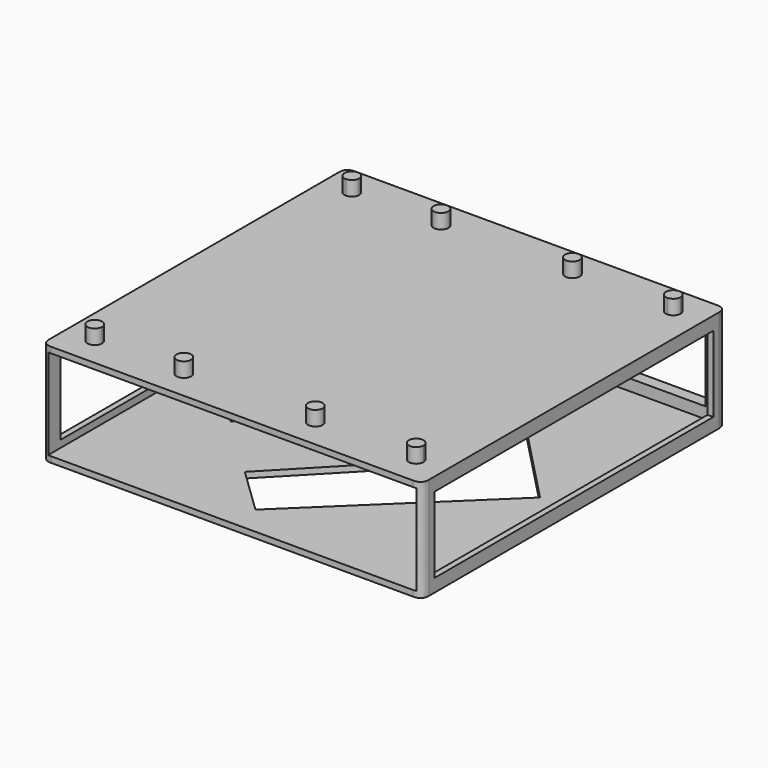
from build123d import *

# Parameters (mm, degrees)
F0_W         = 130
F0_H         = 130
F1_DEPTH     = 17.5
F2_W         = 126
F2_H         = 31
F3_DEPTH     = 126
F5_DEPTH     = 5
F7_DEPTH     = 3
F9_W         = 122.3782406645
F9_H         = 23.2565429012
F10_DEPTH    = 7
F8_W         = 119.2743226562
F8_H         = 26.0036256061
F11_DEPTH    = 130
F12_T1_DEPTH = 50


# Not quite as in the source:
# - a fillet or chamfer that OpenCascade refuses, or shapes differently, is made with other operations: its cross-section is extruded or revolved along the edge and cut away or added


with BuildPart() as f1:
    # F0 (on Top) → F1 (new body, symmetric)
    with BuildSketch(Plane.XY):
        with Locations((2.0031377077, 1.1643140912)):
            Rectangle(F0_W, F0_H)
    extrude(amount=F1_DEPTH, both=True)

    # F2 (on face) → F3 (cut)
    with BuildSketch(Plane.XZ.offset(63.8356859088)):
        with Locations((2.0031377077, 0)):
            Rectangle(F2_W, F2_H)
    extrude(amount=-F3_DEPTH, mode=Mode.SUBTRACT)

    # F4 (on face) → F5 (join)
    with BuildSketch(Plane.XY.offset(17.5)):
        with BuildLine():
            Line((-24.9968622923, -53.8356859088), (-19.9968622923, -53.8356859088))
            ThreePointArc((-19.9968622923, -53.8356859088), (-22.4968622923, -51.3356859088), (-24.9968622923, -53.8356859088))
        make_face()
        with BuildLine():
            ThreePointArc((-24.9968622923, -53.8356859088), (-22.4968622923, -56.3356859088), (-19.9968622923, -53.8356859088))
            Line((-19.9968622923, -53.8356859088), (-24.9968622923, -53.8356859088))
        make_face()
        with BuildLine():
            ThreePointArc((-19.9968622923, 56.1643140912), (-22.4968622923, 58.6643140912), (-24.9968622923, 56.1643140912))
            Line((-24.9968622923, 56.1643140912), (-19.9968622923, 56.1643140912))
        make_face()
        with BuildLine():
            Line((-19.9968622923, 56.1643140912), (-24.9968622923, 56.1643140912))
            ThreePointArc((-24.9968622923, 56.1643140912), (-22.4968622923, 53.6643140912), (-19.9968622923, 56.1643140912))
        make_face()
        with BuildLine():
            Line((20.0031377077, 56.1643140912), (25.0031377077, 56.1643140912))
            ThreePointArc((25.0031377077, 56.1643140912), (22.5031377077, 58.6643140912), (20.0031377077, 56.1643140912))
        make_face()
        with BuildLine():
            ThreePointArc((20.0031377077, 56.1643140912), (22.5031377077, 53.6643140912), (25.0031377077, 56.1643140912))
            Line((25.0031377077, 56.1643140912), (20.0031377077, 56.1643140912))
        make_face()
        with BuildLine():
            Line((25.0031377077, -53.8356859088), (20.0031377077, -53.8356859088))
            ThreePointArc((20.0031377077, -53.8356859088), (22.5031377077, -56.3356859088), (25.0031377077, -53.8356859088))
        make_face()
        with BuildLine():
            ThreePointArc((25.0031377077, -53.8356859088), (22.5031377077, -51.3356859088), (20.0031377077, -53.8356859088))
            Line((20.0031377077, -53.8356859088), (25.0031377077, -53.8356859088))
        make_face()
        with BuildLine():
            ThreePointArc((54.5031400741, 56.1643140912), (55.2365873133, 54.3987711796), (57.0031377077, 53.6677538545))
            Line((57.0031377077, 53.6677538545), (57.0031377077, 56.1643140912))
            Line((57.0031377077, 56.1643140912), (54.5031400741, 56.1643140912))
        make_face()
        with BuildLine():
            Line((57.0031377077, 56.1643140912), (57.0031377077, 53.6677538545))
            ThreePointArc((57.0031377077, 53.6677538545), (58.7709046607, 54.3999869016), (59.5031377077, 56.1677538545))
            ThreePointArc((59.5031377077, 56.1677538545), (57.0014178256, 58.6677532629), (54.5031400741, 56.1643140912))
            Line((54.5031400741, 56.1643140912), (57.0031377077, 56.1643140912))
        make_face()
        with BuildLine():
            ThreePointArc((57.0031377077, -51.3110916167), (55.2314275833, -52.0546307181), (54.51056035, -53.8356859088))
            Line((54.51056035, -53.8356859088), (57.0031377077, -53.8356859088))
            Line((57.0031377077, -53.8356859088), (57.0031377077, -51.3110916167))
        make_face()
        with BuildLine():
            Line((57.0031377077, -53.8356859088), (54.51056035, -53.8356859088))
            ThreePointArc((54.51056035, -53.8356859088), (57.0227418926, -56.311050683), (59.5104392663, -53.8110809541))
            ThreePointArc((59.5104392663, -53.8110809541), (58.7756228408, -52.0407343925), (57.0031377077, -51.3110916167))
            Line((57.0031377077, -51.3110916167), (57.0031377077, -53.8356859088))
        make_face()
        with BuildLine():
            ThreePointArc((-50.4950310388, -53.8363249032), (-50.4950310593, -53.836005406), (-50.4950311205, -53.8356859088))
            Line((-50.4950311205, -53.8356859088), (-52.9968622923, -53.8356859088))
            Line((-52.9968622923, -53.8356859088), (-52.9968622923, -51.3363255739))
            ThreePointArc((-52.9968622923, -51.3363255739), (-54.7621504273, -55.6047391835), (-50.4950310388, -53.8363249032))
        make_face()
        with BuildLine():
            Line((-52.9968622923, -53.8356859088), (-50.4950311205, -53.8356859088))
            ThreePointArc((-50.4950311205, -53.8356859088), (-51.2281376662, -52.0676848015), (-52.9968622923, -51.3363255739))
            Line((-52.9968622923, -51.3363255739), (-52.9968622923, -53.8356859088))
        make_face()
        with BuildLine():
            Line((-52.9968622923, 56.1643140912), (-52.9968622923, 53.6671405204))
            ThreePointArc((-52.9968622923, 53.6671405204), (-51.2364160366, 54.4018236777), (-50.506650387, 56.1643140912))
            Line((-50.506650387, 56.1643140912), (-52.9968622923, 56.1643140912))
        make_face()
        with BuildLine():
            ThreePointArc((-50.5066488108, 56.1671213651), (-54.777872441, 57.9314248684), (-52.9968622923, 53.6671405204))
            Line((-52.9968622923, 53.6671405204), (-52.9968622923, 56.1643140912))
            Line((-52.9968622923, 56.1643140912), (-50.506650387, 56.1643140912))
            ThreePointArc((-50.506650387, 56.1643140912), (-50.5066492049, 56.1657177279), (-50.5066488108, 56.1671213651))
        make_face()
    extrude(amount=F5_DEPTH)

    # F6 (on face) → F7 (cut)
    with BuildSketch(Plane(origin=(0, 0, -17.5), x_dir=(1, 0, 0), z_dir=(0, 0, -1))):
        Polygon((57.0031377077, 0.8356859088), (2.0031377077, 53.8356859088), (-13.8737854376, 38.5361054233), (22.9762229292, 0.2955307031), (-16.0963200722, -37.3561925527), (2.0758649804, -56.1643140912), align=None)
        Polygon((-35.0628468777, 18.1175553083), (-52.9968622923, 0.8356859088), (-36.3205869987, -16.424176437), (-18.4094090927, 0.8356859088), align=None)
    extrude(amount=-F7_DEPTH, mode=Mode.SUBTRACT)

    # F9 (on face) → F10 (cut)
    with BuildSketch(Plane(origin=(0, 66.1643140912, 0), x_dir=(-1, 0, 0), z_dir=(0, 1, 0))):
        with Locations((-2.0031377077, 0)):
            Rectangle(F9_W, F9_H)
    extrude(amount=-F10_DEPTH, mode=Mode.SUBTRACT)

    # F8 (on face) → F11 (cut)
    with BuildSketch(Plane(origin=(-62.9968622923, 0, 0), x_dir=(0, -1, 0), z_dir=(-1, 0, 0))):
        with Locations((-1.2152138836, -0.0606838628)):
            Rectangle(F8_W, F8_H)
    extrude(amount=-F11_DEPTH, mode=Mode.SUBTRACT)

    # F12: fillet of radius 3 on 4 edges, made by hand

    # F12_s2 → F12_t1 (cut)
    with BuildSketch(Plane.XY.offset(-25)):
        with BuildLine():
            add(Edge.make_bspline(
                [(-59.9968622923, 66.1643140912), (-62.9968622923, 66.1643140912), (-62.9968622923, 63.1643140912)],
                knots=[0, 0, 0, 1, 1, 1], degree=2, weights=[1, 1, 1]))
            Line((-62.9968622923, 63.1643140912), (-62.9968622923, 66.1643140912))
            Line((-62.9968622923, 66.1643140912), (-59.9968622923, 66.1643140912))
        make_face()
        with BuildLine():
            add(Edge.make_bspline(
                [(-62.9968622923, -60.8356859088), (-62.9968622923, -63.8356859088), (-59.9968622923, -63.8356859088)],
                knots=[0, 0, 0, 1, 1, 1], degree=2, weights=[1, 1, 1]))
            Line((-59.9968622923, -63.8356859088), (-62.9968622923, -63.8356859088))
            Line((-62.9968622923, -63.8356859088), (-62.9968622923, -60.8356859088))
        make_face()
        with BuildLine():
            add(Edge.make_bspline(
                [(64.0031377077, 66.1643140912), (67.0031377077, 66.1643140912), (67.0031377077, 63.1643140912)],
                knots=[0, 0, 0, 1, 1, 1], degree=2, weights=[1, 1, 1]))
            Line((67.0031377077, 63.1643140912), (67.0031377077, 66.1643140912))
            Line((67.0031377077, 66.1643140912), (64.0031377077, 66.1643140912))
        make_face()
        with BuildLine():
            add(Edge.make_bspline(
                [(67.0031377077, -60.8356859088), (67.0031377077, -63.8356859088), (64.0031377077, -63.8356859088)],
                knots=[0, 0, 0, 1, 1, 1], degree=2, weights=[1, 1, 1]))
            Line((64.0031377077, -63.8356859088), (67.0031377077, -63.8356859088))
            Line((67.0031377077, -63.8356859088), (67.0031377077, -60.8356859088))
        make_face()
    extrude(amount=F12_T1_DEPTH, mode=Mode.SUBTRACT)


solid = f1.part
